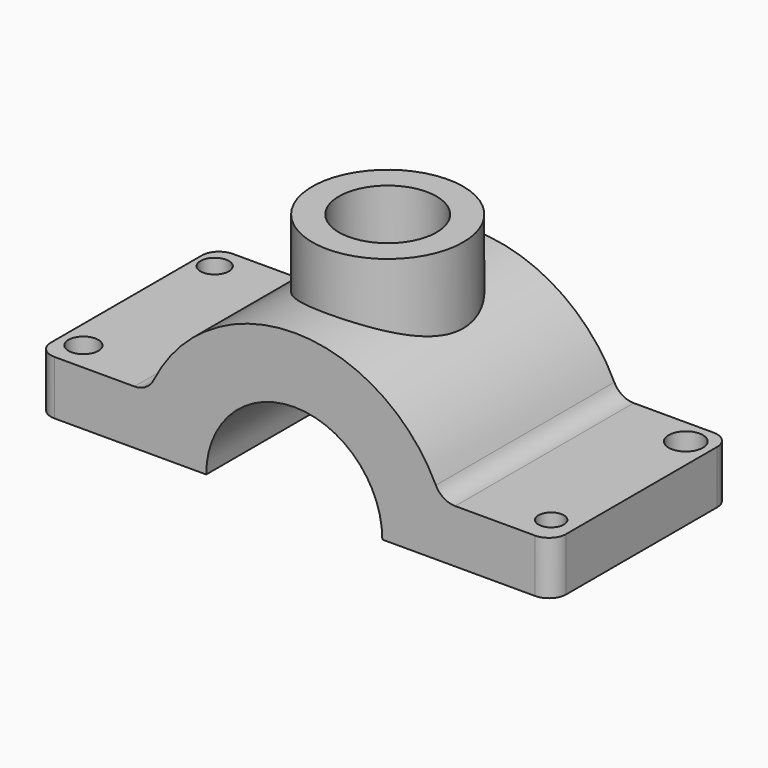
from build123d import *

# Parameters (mm, degrees)
F1_DEPTH  = 65.786
F2_R      = 4.1764569431
F2_R_2    = 4.4090075628
F3_DEPTH  = 25.4
F2_R_3    = 5.0559602499
F2_R_4    = 3.7416125294
F4_DEPTH  = 25.4
F5_R      = 14.3858151817
F6_DEPTH  = 68.072
F5_R_2    = 22.255871479
F7_DEPTH  = 61.976
F8_R      = 5.08
F9_R      = 25.9662767353
F10_DEPTH = 113.792


# Not quite as in the source:
# - a feature names something its author has since deleted; it is built from what else it names


with BuildPart() as f1:
    # F0 (on Front) → F1 (new body)
    with BuildSketch(Plane.XZ):
        with BuildLine():
            ThreePointArc((-25.7879418184, 0), (0, 25.7879418184), (25.7879418184, 0))
            Line((25.7879418184, 0), (76.1246234179, 0))
            Line((76.1246234179, 0), (76.1246234179, 15.6854130328))
            Line((76.1246234179, 15.6854130328), (47.4599736899, 15.6854130328))
            ThreePointArc((47.4599736899, 15.6854130328), (44.0974699454, 16.6487565032), (41.7552011698, 19.2464937988))
            ThreePointArc((41.7552011698, 19.2464937988), (0.2284915035, 45.2565071244), (-41.4557046581, 19.4996400932))
            ThreePointArc((-41.4557046581, 19.4996400932), (-43.7973018606, 16.9263567372), (-47.1434027, 15.9732177854))
            Line((-47.1434027, 15.9732177854), (-75.83681494, 15.9732177854))
            Line((-75.83681494, 15.9732177854), (-75.83681494, 0))
            Line((-75.83681494, 0), (-25.7879418184, 0))
        make_face()
    extrude(amount=F1_DEPTH)

    # F2 (on face) → F3 (cut)
    with BuildSketch(Plane.XY.offset(15.9732177854)):
        with Locations((-70.1924338937, -7.3858876713)):
            Circle(F2_R)
        with Locations((-69.1219046712, -57.112660259)):
            Circle(F2_R_2)
    extrude(amount=-F3_DEPTH, mode=Mode.SUBTRACT)

    # F2 (on face) → F4 (cut)
    with BuildSketch(Plane.XY.offset(15.9732177854)):
        with Locations((68.7799453735, -7.4367355555)):
            Circle(F2_R_3)
        with Locations((69.0292343497, -57.3799200356)):
            Circle(F2_R_4)
    extrude(amount=-F4_DEPTH, mode=Mode.SUBTRACT)

    # F5 (on Top) → F6 (cut)
    with BuildSketch(Plane.XY):
        with Locations((0, -31.3370935619)):
            Circle(F5_R)
    extrude(amount=F6_DEPTH, mode=Mode.SUBTRACT)

    # F5 (on Top) → F7 (join)
    with BuildSketch(Plane.XY):
        with Locations((0, -31.3370935619)):
            Circle(F5_R_2)
        with Locations((0, -31.3370935619)):
            Circle(F5_R, mode=Mode.SUBTRACT)
    extrude(amount=F7_DEPTH)

    # F8
    f8_edges = [f1.edges().sort_by_distance(p)[0] for p in [
        (76.124623, -65.786, 7.842707),
        (76.124623, 0, 7.842707),
        (-75.836815, 0, 7.986609),
        (-75.836815, -65.786, 7.986609),
    ]]
    fillet(f8_edges, radius=F8_R)

    # F9 (on Front) → F10 (cut)
    with BuildSketch(Plane.XZ):
        Circle(F9_R)
    extrude(amount=F10_DEPTH, mode=Mode.SUBTRACT)


solid = f1.part
